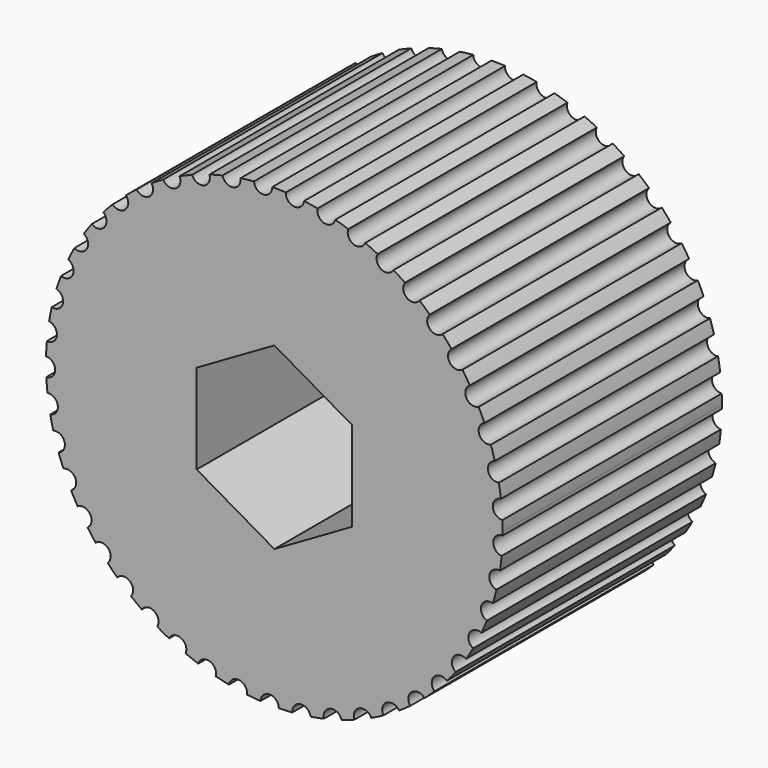
from build123d import *

# Parameters (mm, degrees)
F0_R     = 12.5
F0_R_2   = 5
F1_DEPTH = 15
F2_DEPTH = 15
F0_R_3   = 2.75
F3_DEPTH = 5
F4_DEPTH = 3
F5_DEPTH = 3
F7_R     = 0.5
F8_DEPTH = 15


# Not quite as in the source:
# - a fillet or chamfer that OpenCascade refuses, or shapes differently, is made with other operations: its cross-section is extruded or revolved along the edge and cut away or added


with BuildPart() as f1:
    # F0 (on Front) → F1 (new body)
    with BuildSketch(Plane.XZ):
        Circle(F0_R)
        Circle(F0_R_2, mode=Mode.SUBTRACT)
    extrude(amount=F1_DEPTH)

    # F0 (on Front) → F2 (join)
    with BuildSketch(Plane.XZ):
        Circle(F0_R_2)
        Polygon((-4.2491954474, -2.4551316428), (-4.250804096, 2.4523453817), (-0.0016086486, 4.9074770245), (4.2491954474, 2.4551316428), (4.250804096, -2.4523453817), (0.0016086486, -4.9074770245), align=None, mode=Mode.SUBTRACT)
    extrude(amount=F2_DEPTH)

    # F0 (on Front) → F3 (join)
    with BuildSketch(Plane.XZ):
        Polygon((-0.0016086486, 4.9074770245), (-4.250804096, 2.4523453817), (-4.2491954474, -2.4551316428), (0.0016086486, -4.9074770245), (4.250804096, -2.4523453817), (4.2491954474, 2.4551316428), align=None)
        Circle(F0_R_3, mode=Mode.SUBTRACT)
    extrude(amount=F3_DEPTH)

    # F0 (on Front) → F4 (join)
    with BuildSketch(Plane.XZ):
        Circle(F0_R_2)
        Polygon((-4.2491954474, -2.4551316428), (-4.250804096, 2.4523453817), (-0.0016086486, 4.9074770245), (4.2491954474, 2.4551316428), (4.250804096, -2.4523453817), (0.0016086486, -4.9074770245), align=None, mode=Mode.SUBTRACT)
    extrude(amount=-F4_DEPTH)

    # F0 (on Front) → F5 (join)
    with BuildSketch(Plane.XZ):
        Polygon((-0.0016086486, 4.9074770245), (-4.250804096, 2.4523453817), (-4.2491954474, -2.4551316428), (0.0016086486, -4.9074770245), (4.250804096, -2.4523453817), (4.2491954474, 2.4551316428), align=None)
        Circle(F0_R_3, mode=Mode.SUBTRACT)
    extrude(amount=-F5_DEPTH)

    # F6: chamfer of 2.5 on 1 edges, made by hand

    # F6_s1 → F6_t2 (revolve, cut)
    with BuildSketch(Plane.XY):
        Polygon((2.5, 3), (5, 0.5), (5, 3), align=None)
    revolve(axis=Axis((0, 3, 0), (0, -1, 0)), mode=Mode.SUBTRACT)

    # F7 (on Front) → F8 (cut)
    with BuildSketch(Plane.XZ):
        with Locations((-5.3183648548, -11.3121613881)):
            Circle(F7_R)
        with Locations((-3.6922583147, -11.94224554)):
            Circle(F7_R)
        with Locations((-1.9942861663, -12.3398874665)):
            Circle(F7_R)
        with Locations((-0.2574975062, -12.4973475199)):
            Circle(F7_R)
        with Locations((1.4843030499, -12.4115609194)):
            Circle(F7_R)
        with Locations((3.1972133356, -12.0841974035)):
            Circle(F7_R)
        with Locations((4.8478935004, -11.5216287307)):
            Circle(F7_R)
        with Locations((6.4042149327, -10.7348046603)):
            Circle(F7_R)
        with Locations((7.835885606, -9.7390398279)):
            Circle(F7_R)
        with Locations((9.1150396792, -8.5537156632)):
            Circle(F7_R)
        with Locations((10.2167798732, -7.2019031529)):
            Circle(F7_R)
        with Locations((11.1196620684, -5.7099137897)):
            Circle(F7_R)
        with Locations((11.8061126898, -4.1067874495)):
            Circle(F7_R)
        with Locations((12.262770757, -2.423727163)):
            Circle(F7_R)
        with Locations((12.4807479401, -0.6934917843)):
            Circle(F7_R)
        with Locations((12.4558015612, 1.0502416232)):
            Circle(F7_R)
        with Locations((12.1884171732, 2.7735332722)):
            Circle(F7_R)
        with Locations((11.683799109, 4.4428412508)):
            Circle(F7_R)
        with Locations((10.9517691853, 6.0256743782)):
            Circle(F7_R)
        with Locations((10.0065755319, 7.4912246078)):
            Circle(F7_R)
        with Locations((8.866615268, 8.8109666717)):
            Circle(F7_R)
        with Locations((7.5540764236, 9.9592132916)):
            Circle(F7_R)
        with Locations((6.0945060742, 10.9136151532)):
            Circle(F7_R)
        with Locations((4.5163130964, 11.6555959099)):
            Circle(F7_R)
        with Locations((2.8502152215, 12.1707137503)):
            Circle(F7_R)
        with Locations((1.1286411494, 12.4489424915)):
            Circle(F7_R)
        with Locations((-0.6149006389, 12.4848667275)):
            Circle(F7_R)
        with Locations((-2.3464740857, 12.2777872341)):
            Circle(F7_R)
        with Locations((-4.0323760835, 11.8317345779)):
            Circle(F7_R)
        with Locations((-5.6397924676, 11.1553906665)):
            Circle(F7_R)
        with Locations((-7.1374367064, 10.2619197649)):
            Circle(F7_R)
        with Locations((-8.4961588585, 9.1687122678)):
            Circle(F7_R)
        with Locations((-9.6895129427, 7.8970462157)):
            Circle(F7_R)
        with Locations((-10.6942716791, 6.4716731418)):
            Circle(F7_R)
        with Locations((-11.4908785818, 4.9203363116)):
            Circle(F7_R)
        with Locations((-12.0638286036, 3.2732307318)):
            Circle(F7_R)
        with Locations((-12.401969924, 1.5624154391)):
            Circle(F7_R)
        with Locations((-12.4987210069, -0.1788104928)):
            Circle(F7_R)
        with Locations((-12.3521987024, -1.916556082)):
            Circle(F7_R)
        with Locations((-11.9652549007, -3.616998087)):
            Circle(F7_R)
        with Locations((-11.3454210226, -5.2470393386)):
            Circle(F7_R)
        with Locations((-10.5047614295, -6.7749529378)):
            Circle(F7_R)
        with Locations((-9.4596386041, -8.1709997846)):
            Circle(F7_R)
        with Locations((-8.2303946735, -9.4080074148)):
            Circle(F7_R)
        with Locations((-6.8409554726, -10.4618988822)):
            Circle(F7_R)
    extrude(amount=F8_DEPTH, mode=Mode.SUBTRACT)


solid = f1.part
